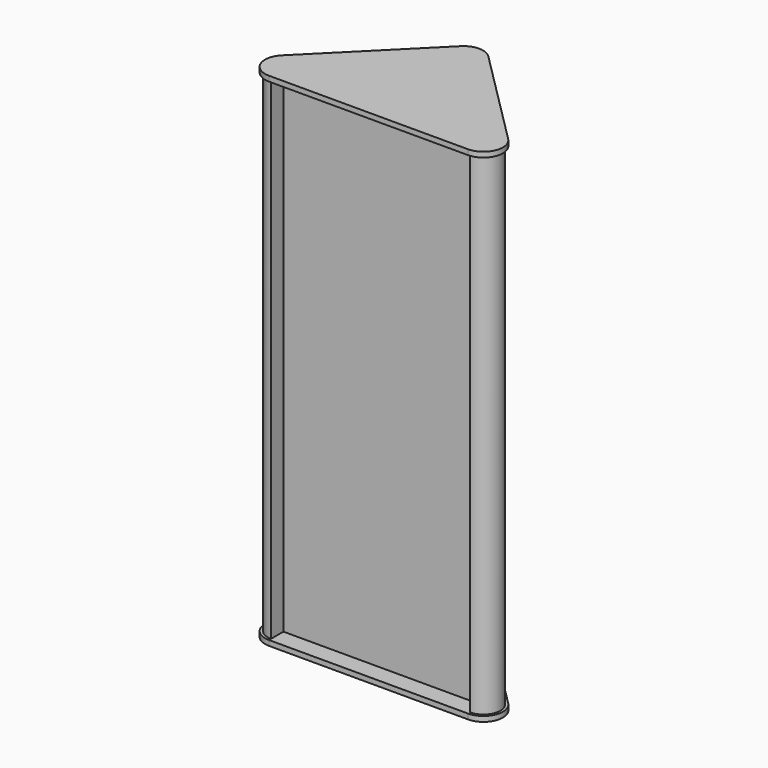
from build123d import *

# Parameters (mm, degrees)
F1_DEPTH    = 4
F2_R        = 15
F4_DEPTH    = 380
F5_T1_DEPTH = 458.4619407771
F5_T3_DEPTH = 412.5
F7_DEPTH    = 4
F8_R        = 15
F9_W        = 153.8477631085
F9_H        = 380
F10_DEPTH   = 12


# Not quite as in the source:
# - a fillet or chamfer that OpenCascade refuses, or shapes differently, is made with other operations: its cross-section is extruded or revolved along the edge and cut away or added


with BuildPart() as f1:
    # F0 (on Top) → F1 (new body)
    with BuildSketch(Plane.XY):
        Polygon((0, 63.1370849898), (-113.1370849898, -50), (113.1370849898, -50), align=None)
    extrude(amount=F1_DEPTH)

    # F2
    f2_edges = [f1.edges().sort_by_distance(p)[0] for p in [
        (-113.137085, -50, 2),
        (113.137085, -50, 2),
        (0, 63.137085, 2),
    ]]
    fillet(f2_edges, radius=F2_R)

    # F3 (on face) → F4 (join)
    with BuildSketch(Plane.XY.offset(4)):
        Polygon((108.3086578651, -48), (0, 60.3086578651), (-108.3086578651, -48), align=None)
    extrude(amount=F4_DEPTH)

    # F5: fillet of radius 13 on 3 edges, made by hand

    # F5_s2 → F5_t1 (cut)
    with BuildSketch(Plane.XY.offset(4)):
        with BuildLine():
            ThreePointArc((86.1162697097, -25.8076118446), (88.9343154769, -39.9748846207), (76.9238815543, -48))
            Line((76.9238815543, -48), (108.3086578651, -48))
            Line((108.3086578651, -48), (86.1162697097, -25.8076118446))
        make_face()
        with BuildLine():
            ThreePointArc((-86.1162697097, -25.8076118446), (-88.9343154769, -39.9748846207), (-76.9238815543, -48))
            Line((-76.9238815543, -48), (-108.3086578651, -48))
            Line((-108.3086578651, -48), (-86.1162697097, -25.8076118446))
        make_face()
    extrude(amount=F5_T1_DEPTH, mode=Mode.SUBTRACT)

    # F5_s4 → F5_t3 (cut)
    with BuildSketch(Plane.XY.offset(4)):
        with BuildLine():
            ThreePointArc((-9.1923881554, 51.1162697097), (0, 54.9238815543), (9.1923881554, 51.1162697097))
            Line((9.1923881554, 51.1162697097), (0, 60.3086578651))
            Line((0, 60.3086578651), (-9.1923881554, 51.1162697097))
        make_face()
    extrude(amount=F5_T3_DEPTH, mode=Mode.SUBTRACT)

    # F6 (on face) → F7 (join)
    with BuildSketch(Plane.XY.offset(384)):
        Polygon((0, 63.1370849898), (-113.1370849898, -50), (113.1370849898, -50), align=None)
    extrude(amount=F7_DEPTH)

    # F8
    f8_edges = [f1.edges().sort_by_distance(p)[0] for p in [
        (113.137085, -50, 386),
        (-113.137085, -50, 386),
        (0, 63.137085, 386),
    ]]
    fillet(f8_edges, radius=F8_R)

    # F9 (on face) → F10 (cut)
    with BuildSketch(Plane.XZ.offset(48)):
        with Locations((0, 194)):
            Rectangle(F9_W, F9_H)
    extrude(amount=-F10_DEPTH, mode=Mode.SUBTRACT)


solid = f1.part
